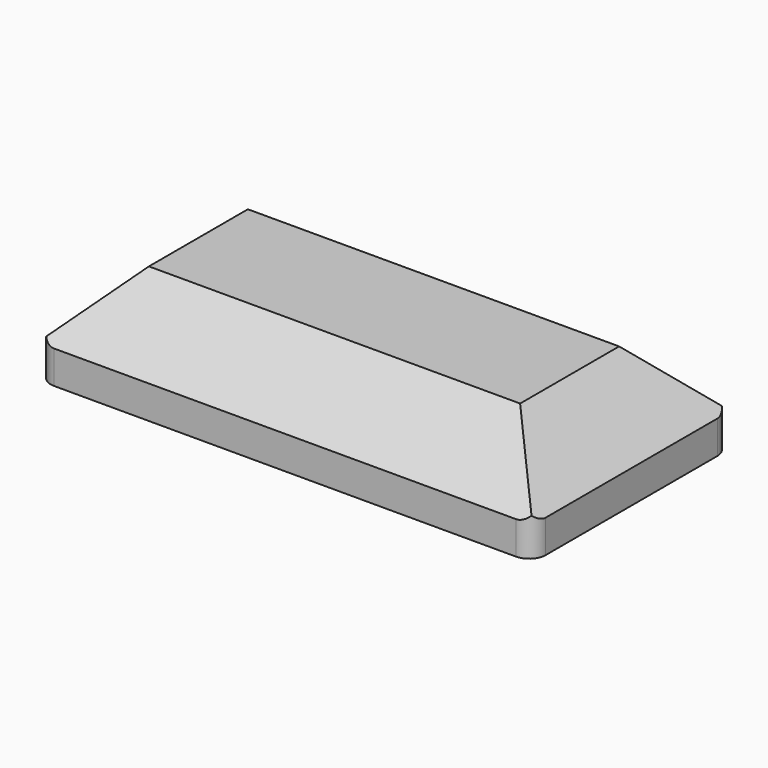
from build123d import *

# Parameters (mm, degrees)
F0_W     = 152.4
F0_H     = 76.2
F1_DEPTH = 19.05
F2_SIZE  = 19.04999
F3_W     = 152.4
F3_H     = 76.2
F4_DEPTH = 10.16
F5_T     = -2.032
F6_R     = 5.08


# Not quite as in the source:
# - a fillet or chamfer is up to 0.001 mm smaller than in the source, because OpenCascade refuses the exact size


with BuildPart() as f1:
    # F0 (on Top) → F1 (new body)
    with BuildSketch(Plane.XY):
        with Locations((-76.2, -38.1)):
            Rectangle(F0_W, F0_H)
    extrude(amount=F1_DEPTH)

    # F2 (size 19.05 in the source; OpenCascade refuses exactly that, so slightly less here)
    f2_edges = [f1.edges().sort_by_distance(p)[0] for p in [
        (0, -38.1, 19.05),
        (-76.2, 0, 19.05),
        (-152.4, -38.1, 19.05),
        (-76.2, -76.2, 19.05),
    ]]
    chamfer(f2_edges, length=F2_SIZE)

    # F3 (on face) → F4 (join)
    with BuildSketch(Plane(origin=(0, 0, 0), x_dir=(1, 0, 0), z_dir=(0, 0, -1))):
        with Locations((-76.2, 38.1)):
            Rectangle(F3_W, F3_H)
    extrude(amount=F4_DEPTH)

    # F5
    f5_openings = [f1.faces().sort_by_distance(p)[0] for p in [
        (-76.2, -38.1, -10.16),
    ]]
    offset(amount=F5_T, openings=f5_openings)

    # F6
    f6_edges = [f1.edges().sort_by_distance(p)[0] for p in [
        (0, 0, -5.08),
        (-152.4, 0, -5.08),
        (-152.4, -76.2, -5.08),
        (0, -76.2, -5.08),
    ]]
    fillet(f6_edges, radius=F6_R)


solid = f1.part
